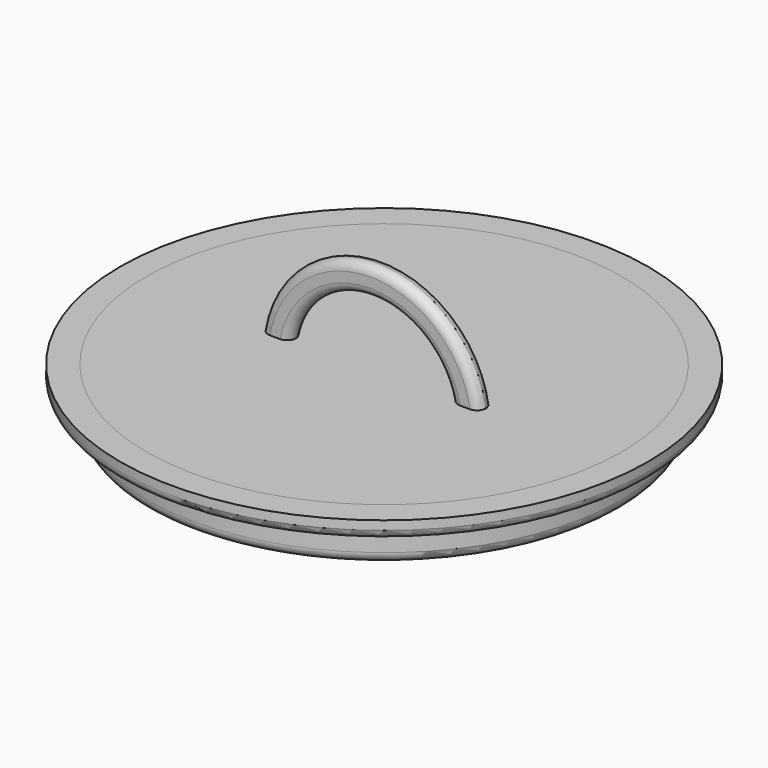
from build123d import *

# Parameters (mm, degrees)
F0_R      = 38.1
F0_R_2    = 34.29
F1_DEPTH  = 2.54
F2_R      = 1.27
F3_R      = 15.9349735513
F3_R_2    = 11.9674764151
F4_DEPTH  = 2.54
F5_R      = 1.26999
F6_DEPTH  = 5.08
F7_DEPTH  = 2.54
F8_R      = 1.524
F9_W      = 32.174937427
F9_H      = 8.878018707
F10_DEPTH = 17.2739680856


# Not quite as in the source:
# - a fillet or chamfer is up to 0.001 mm smaller than in the source, because OpenCascade refuses the exact size


with BuildPart() as f1:
    # F0 (on Top) → F1 (new body)
    with BuildSketch(Plane.XY):
        Circle(F0_R)
        Circle(F0_R_2, mode=Mode.SUBTRACT)
    extrude(amount=F1_DEPTH)

    # F2
    f2_edges = [f1.edges().sort_by_distance(p)[0] for p in [
        (-38.1, 0, 0),
    ]]
    fillet(f2_edges, radius=F2_R)


with BuildPart() as f4:
    # F3 (on Front) → F4 (new body)
    with BuildSketch(Plane.XZ):
        Circle(F3_R)
        Circle(F3_R_2, mode=Mode.SUBTRACT)
    extrude(amount=F4_DEPTH)

    # F5 (radius 1.27 in the source; OpenCascade refuses exactly that, so slightly less here)
    f5_edges = [f4.edges().sort_by_distance(p)[0] for p in [
        (-15.934974, -2.54, 0),
        (-11.967476, 0, 0),
        (-15.934974, 0, 0),
        (-11.967476, -2.54, 0),
    ]]
    fillet(f5_edges, radius=F5_R)

    # F9 (on face) → F10 (cut)
    with BuildSketch(Plane(origin=(0, 0, -5.08), x_dir=(1, 0, 0), z_dir=(0, 0, -1))):
        with Locations((0.0944472849, 1.2278128415)):
            Rectangle(F9_W, F9_H)
    extrude(amount=F10_DEPTH, mode=Mode.SUBTRACT)


with BuildPart() as f6:
    # F0 (on Top) → F6 (new body)
    with BuildSketch(Plane.XY):
        Circle(F0_R_2)
    extrude(amount=-F6_DEPTH)

    # F8
    f8_edges = [f6.edges().sort_by_distance(p)[0] for p in [
        (-34.29, 0, -5.08),
    ]]
    fillet(f8_edges, radius=F8_R)


with BuildPart() as f7:
    # F0 (on Top) → F7 (new body)
    with BuildSketch(Plane.XY):
        Circle(F0_R_2)
    extrude(amount=F7_DEPTH)


solid = Compound([f1.part, f4.part, f6.part, f7.part])
